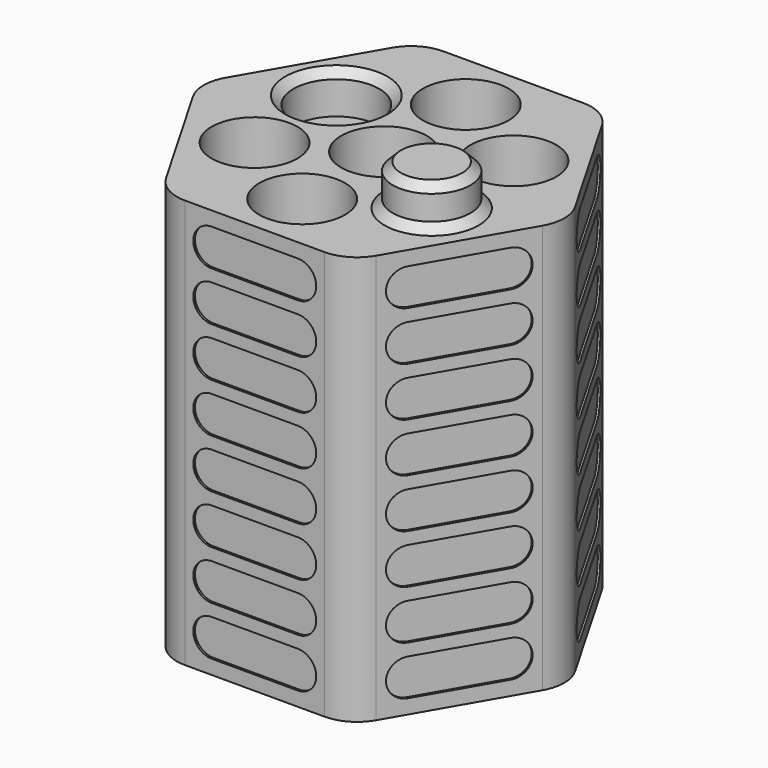
from build123d import *

# Parameters (mm, degrees)
F0_R      = 5.25
F0_R_2    = 4.75
F1_DEPTH  = 50
F2_DEPTH  = 5
F3_DEPTH  = 55
F4_DEPTH  = 45
F5_SIZE   = 1
F6_R      = 5
F8_DEPTH  = 0.25
F10_DEPTH = 0.25
F12_DEPTH = 0.25
F14_DEPTH = 0.25
F16_DEPTH = 0.25
F18_DEPTH = 0.25


with BuildPart() as f1:
    # F0 (on Top) → F1 (new body)
    with BuildSketch(Plane.XY):
        Polygon((11.4026678165, 19.75), (-11.4026678165, 19.75), (-22.805335633, 0), (-11.4026678165, -19.75), (11.4026678165, -19.75), (22.805335633, 0), align=None)
        with Locations((-10.8253175473, -6.25)):
            Circle(F0_R, mode=Mode.SUBTRACT)
        with Locations((0, -12.5)):
            Circle(F0_R, mode=Mode.SUBTRACT)
        with Locations((10.8253175473, -6.25)):
            Circle(F0_R_2, mode=Mode.SUBTRACT)
        with Locations((-10.8253175473, 6.25)):
            Circle(F0_R, mode=Mode.SUBTRACT)
        Circle(F0_R, mode=Mode.SUBTRACT)
        with Locations((10.8253175473, 6.25)):
            Circle(F0_R, mode=Mode.SUBTRACT)
        with Locations((0, 12.5)):
            Circle(F0_R, mode=Mode.SUBTRACT)
    extrude(amount=F1_DEPTH)

    # F0 (on Top) → F2 (join)
    with BuildSketch(Plane.XY):
        Circle(F0_R)
        with Locations((0, 12.5)):
            Circle(F0_R)
        with Locations((-10.8253175473, -6.25)):
            Circle(F0_R)
        with Locations((0, -12.5)):
            Circle(F0_R)
        with Locations((10.8253175473, 6.25)):
            Circle(F0_R)
    extrude(amount=F2_DEPTH)

    # F0 (on Top) → F3 (join)
    with BuildSketch(Plane.XY):
        with Locations((10.8253175473, -6.25)):
            Circle(F0_R_2)
    extrude(amount=F3_DEPTH)

    # F0 (on Top) → F4 (join)
    with BuildSketch(Plane.XY):
        with Locations((-10.8253175473, 6.25)):
            Circle(F0_R)
    extrude(amount=F4_DEPTH)

    # F5
    f5_edges = [f1.edges().sort_by_distance(p)[0] for p in [
        (6.075318, -6.25, 55),
        (-16.075318, 6.25, 50),
        (6.075318, -6.25, 50),
    ]]
    chamfer(f5_edges, length=F5_SIZE)

    # F6
    f6_edges = [f1.edges().sort_by_distance(p)[0] for p in [
        (22.805336, 0, 25),
        (11.402668, 19.75, 25),
        (-11.402668, 19.75, 25),
        (-22.805336, 0, 25),
        (-11.402668, -19.75, 25),
        (11.402668, -19.75, 25),
    ]]
    fillet(f6_edges, radius=F6_R)

    # F7 (on face) → F8 (cut)
    with BuildSketch(Plane.XZ.offset(19.75)):
        with BuildLine():
            Line((5.2659164705, 48.25), (-5.2659164705, 48.25))
            ThreePointArc((-5.2659164705, 48.25), (-7.5159164705, 46), (-5.2659164705, 43.75))
            Line((-5.2659164705, 43.75), (5.2659164705, 43.75))
            ThreePointArc((5.2659164705, 43.75), (7.5159164705, 46), (5.2659164705, 48.25))
        make_face()
        with BuildLine():
            Line((5.2659164705, 42.25), (-5.2659164705, 42.25))
            ThreePointArc((-5.2659164705, 42.25), (-7.5159164705, 40), (-5.2659164705, 37.75))
            Line((-5.2659164705, 37.75), (5.2659164705, 37.75))
            ThreePointArc((5.2659164705, 37.75), (7.5159164705, 40), (5.2659164705, 42.25))
        make_face()
        with BuildLine():
            Line((5.2659164705, 36.25), (-5.2659164705, 36.25))
            ThreePointArc((-5.2659164705, 36.25), (-7.5159164705, 34), (-5.2659164705, 31.75))
            Line((-5.2659164705, 31.75), (5.2659164705, 31.75))
            ThreePointArc((5.2659164705, 31.75), (7.5159164705, 34), (5.2659164705, 36.25))
        make_face()
        with BuildLine():
            Line((5.2659164705, 30.25), (-5.2659164705, 30.25))
            ThreePointArc((-5.2659164705, 30.25), (-7.5159164705, 28), (-5.2659164705, 25.75))
            Line((-5.2659164705, 25.75), (5.2659164705, 25.75))
            ThreePointArc((5.2659164705, 25.75), (7.5159164705, 28), (5.2659164705, 30.25))
        make_face()
        with BuildLine():
            Line((5.2659164705, 24.25), (-5.2659164705, 24.25))
            ThreePointArc((-5.2659164705, 24.25), (-7.5159164705, 22), (-5.2659164705, 19.75))
            Line((-5.2659164705, 19.75), (5.2659164705, 19.75))
            ThreePointArc((5.2659164705, 19.75), (7.5159164705, 22), (5.2659164705, 24.25))
        make_face()
        with BuildLine():
            Line((5.2659164705, 18.25), (-5.2659164705, 18.25))
            ThreePointArc((-5.2659164705, 18.25), (-7.5159164705, 16), (-5.2659164705, 13.75))
            Line((-5.2659164705, 13.75), (5.2659164705, 13.75))
            ThreePointArc((5.2659164705, 13.75), (7.5159164705, 16), (5.2659164705, 18.25))
        make_face()
        with BuildLine():
            Line((5.2659164705, 12.25), (-5.2659164705, 12.25))
            ThreePointArc((-5.2659164705, 12.25), (-7.5159164705, 10), (-5.2659164705, 7.75))
            Line((-5.2659164705, 7.75), (5.2659164705, 7.75))
            ThreePointArc((5.2659164705, 7.75), (7.5159164705, 10), (5.2659164705, 12.25))
        make_face()
        with BuildLine():
            Line((5.2659164705, 6.25), (-5.2659164705, 6.25))
            ThreePointArc((-5.2659164705, 6.25), (-7.5159164705, 4), (-5.2659164705, 1.75))
            Line((-5.2659164705, 1.75), (5.2659164705, 1.75))
            ThreePointArc((5.2659164705, 1.75), (7.5159164705, 4), (5.2659164705, 6.25))
        make_face()
    extrude(amount=-F8_DEPTH, mode=Mode.SUBTRACT)

    # F9 (on face) → F10 (cut)
    with BuildSketch(Plane(origin=(17.1040017247, -9.875, 0), x_dir=(0.5, 0.8660254038, 0), z_dir=(0.8660254038, -0.5, 0))):
        with BuildLine():
            Line((5.2659164705, 48.25), (-5.2659164705, 48.25))
            ThreePointArc((-5.2659164705, 48.25), (-7.5159164705, 46), (-5.2659164705, 43.75))
            Line((-5.2659164705, 43.75), (5.2659164705, 43.75))
            ThreePointArc((5.2659164705, 43.75), (7.5159164705, 46), (5.2659164705, 48.25))
        make_face()
        with BuildLine():
            Line((5.2659164705, 42.25), (-5.2659164705, 42.25))
            ThreePointArc((-5.2659164705, 42.25), (-7.5159164705, 40), (-5.2659164705, 37.75))
            Line((-5.2659164705, 37.75), (5.2659164705, 37.75))
            ThreePointArc((5.2659164705, 37.75), (7.5159164705, 40), (5.2659164705, 42.25))
        make_face()
        with BuildLine():
            Line((5.2659164705, 36.25), (-5.2659164705, 36.25))
            ThreePointArc((-5.2659164705, 36.25), (-7.5159164705, 34), (-5.2659164705, 31.75))
            Line((-5.2659164705, 31.75), (5.2659164705, 31.75))
            ThreePointArc((5.2659164705, 31.75), (7.5159164705, 34), (5.2659164705, 36.25))
        make_face()
        with BuildLine():
            Line((5.2659164705, 30.25), (-5.2659164705, 30.25))
            ThreePointArc((-5.2659164705, 30.25), (-7.5159164705, 28), (-5.2659164705, 25.75))
            Line((-5.2659164705, 25.75), (5.2659164705, 25.75))
            ThreePointArc((5.2659164705, 25.75), (7.5159164705, 28), (5.2659164705, 30.25))
        make_face()
        with BuildLine():
            Line((5.2659164705, 24.25), (-5.2659164705, 24.25))
            ThreePointArc((-5.2659164705, 24.25), (-7.5159164705, 22), (-5.2659164705, 19.75))
            Line((-5.2659164705, 19.75), (5.2659164705, 19.75))
            ThreePointArc((5.2659164705, 19.75), (7.5159164705, 22), (5.2659164705, 24.25))
        make_face()
        with BuildLine():
            Line((5.2659164705, 18.25), (-5.2659164705, 18.25))
            ThreePointArc((-5.2659164705, 18.25), (-7.5159164705, 16), (-5.2659164705, 13.75))
            Line((-5.2659164705, 13.75), (5.2659164705, 13.75))
            ThreePointArc((5.2659164705, 13.75), (7.5159164705, 16), (5.2659164705, 18.25))
        make_face()
        with BuildLine():
            Line((5.2659164705, 12.25), (-5.2659164705, 12.25))
            ThreePointArc((-5.2659164705, 12.25), (-7.5159164705, 10), (-5.2659164705, 7.75))
            Line((-5.2659164705, 7.75), (5.2659164705, 7.75))
            ThreePointArc((5.2659164705, 7.75), (7.5159164705, 10), (5.2659164705, 12.25))
        make_face()
        with BuildLine():
            Line((5.2659164705, 6.25), (-5.2659164705, 6.25))
            ThreePointArc((-5.2659164705, 6.25), (-7.5159164705, 4), (-5.2659164705, 1.75))
            Line((-5.2659164705, 1.75), (5.2659164705, 1.75))
            ThreePointArc((5.2659164705, 1.75), (7.5159164705, 4), (5.2659164705, 6.25))
        make_face()
    extrude(amount=-F10_DEPTH, mode=Mode.SUBTRACT)

    # F11 (on face) → F12 (cut)
    with BuildSketch(Plane(origin=(17.1040017247, 9.875, 0), x_dir=(-0.5, 0.8660254038, 0), z_dir=(0.8660254038, 0.5, 0))):
        with BuildLine():
            Line((5.2659164705, 48.25), (-5.2659164705, 48.25))
            ThreePointArc((-5.2659164705, 48.25), (-7.5159164705, 46), (-5.2659164705, 43.75))
            Line((-5.2659164705, 43.75), (5.2659164705, 43.75))
            ThreePointArc((5.2659164705, 43.75), (7.5159164705, 46), (5.2659164705, 48.25))
        make_face()
        with BuildLine():
            Line((5.2659164705, 42.25), (-5.2659164705, 42.25))
            ThreePointArc((-5.2659164705, 42.25), (-7.5159164705, 40), (-5.2659164705, 37.75))
            Line((-5.2659164705, 37.75), (5.2659164705, 37.75))
            ThreePointArc((5.2659164705, 37.75), (7.5159164705, 40), (5.2659164705, 42.25))
        make_face()
        with BuildLine():
            Line((5.2659164705, 36.25), (-5.2659164705, 36.25))
            ThreePointArc((-5.2659164705, 36.25), (-7.5159164705, 34), (-5.2659164705, 31.75))
            Line((-5.2659164705, 31.75), (5.2659164705, 31.75))
            ThreePointArc((5.2659164705, 31.75), (7.5159164705, 34), (5.2659164705, 36.25))
        make_face()
        with BuildLine():
            Line((5.2659164705, 30.25), (-5.2659164705, 30.25))
            ThreePointArc((-5.2659164705, 30.25), (-7.5159164705, 28), (-5.2659164705, 25.75))
            Line((-5.2659164705, 25.75), (5.2659164705, 25.75))
            ThreePointArc((5.2659164705, 25.75), (7.5159164705, 28), (5.2659164705, 30.25))
        make_face()
        with BuildLine():
            Line((5.2659164705, 24.25), (-5.2659164705, 24.25))
            ThreePointArc((-5.2659164705, 24.25), (-7.5159164705, 22), (-5.2659164705, 19.75))
            Line((-5.2659164705, 19.75), (5.2659164705, 19.75))
            ThreePointArc((5.2659164705, 19.75), (7.5159164705, 22), (5.2659164705, 24.25))
        make_face()
        with BuildLine():
            Line((5.2659164705, 18.25), (-5.2659164705, 18.25))
            ThreePointArc((-5.2659164705, 18.25), (-7.5159164705, 16), (-5.2659164705, 13.75))
            Line((-5.2659164705, 13.75), (5.2659164705, 13.75))
            ThreePointArc((5.2659164705, 13.75), (7.5159164705, 16), (5.2659164705, 18.25))
        make_face()
        with BuildLine():
            Line((5.2659164705, 12.25), (-5.2659164705, 12.25))
            ThreePointArc((-5.2659164705, 12.25), (-7.5159164705, 10), (-5.2659164705, 7.75))
            Line((-5.2659164705, 7.75), (5.2659164705, 7.75))
            ThreePointArc((5.2659164705, 7.75), (7.5159164705, 10), (5.2659164705, 12.25))
        make_face()
        with BuildLine():
            Line((5.2659164705, 6.25), (-5.2659164705, 6.25))
            ThreePointArc((-5.2659164705, 6.25), (-7.5159164705, 4), (-5.2659164705, 1.75))
            Line((-5.2659164705, 1.75), (5.2659164705, 1.75))
            ThreePointArc((5.2659164705, 1.75), (7.5159164705, 4), (5.2659164705, 6.25))
        make_face()
    extrude(amount=-F12_DEPTH, mode=Mode.SUBTRACT)

    # F13 (on face) → F14 (cut)
    with BuildSketch(Plane(origin=(0, 19.75, 0), x_dir=(-1, 0, 0), z_dir=(0, 1, 0))):
        with BuildLine():
            Line((5.2659164705, 48.25), (-5.2659164705, 48.25))
            ThreePointArc((-5.2659164705, 48.25), (-7.5159164705, 46), (-5.2659164705, 43.75))
            Line((-5.2659164705, 43.75), (5.2659164705, 43.75))
            ThreePointArc((5.2659164705, 43.75), (7.5159164705, 46), (5.2659164705, 48.25))
        make_face()
        with BuildLine():
            Line((5.2659164705, 42.25), (-5.2659164705, 42.25))
            ThreePointArc((-5.2659164705, 42.25), (-7.5159164705, 40), (-5.2659164705, 37.75))
            Line((-5.2659164705, 37.75), (5.2659164705, 37.75))
            ThreePointArc((5.2659164705, 37.75), (7.5159164705, 40), (5.2659164705, 42.25))
        make_face()
        with BuildLine():
            Line((5.2659164705, 36.25), (-5.2659164705, 36.25))
            ThreePointArc((-5.2659164705, 36.25), (-7.5159164705, 34), (-5.2659164705, 31.75))
            Line((-5.2659164705, 31.75), (5.2659164705, 31.75))
            ThreePointArc((5.2659164705, 31.75), (7.5159164705, 34), (5.2659164705, 36.25))
        make_face()
        with BuildLine():
            Line((5.2659164705, 30.25), (-5.2659164705, 30.25))
            ThreePointArc((-5.2659164705, 30.25), (-7.5159164705, 28), (-5.2659164705, 25.75))
            Line((-5.2659164705, 25.75), (5.2659164705, 25.75))
            ThreePointArc((5.2659164705, 25.75), (7.5159164705, 28), (5.2659164705, 30.25))
        make_face()
        with BuildLine():
            Line((5.2659164705, 24.25), (-5.2659164705, 24.25))
            ThreePointArc((-5.2659164705, 24.25), (-7.5159164705, 22), (-5.2659164705, 19.75))
            Line((-5.2659164705, 19.75), (5.2659164705, 19.75))
            ThreePointArc((5.2659164705, 19.75), (7.5159164705, 22), (5.2659164705, 24.25))
        make_face()
        with BuildLine():
            Line((5.2659164705, 18.25), (-5.2659164705, 18.25))
            ThreePointArc((-5.2659164705, 18.25), (-7.5159164705, 16), (-5.2659164705, 13.75))
            Line((-5.2659164705, 13.75), (5.2659164705, 13.75))
            ThreePointArc((5.2659164705, 13.75), (7.5159164705, 16), (5.2659164705, 18.25))
        make_face()
        with BuildLine():
            Line((5.2659164705, 12.25), (-5.2659164705, 12.25))
            ThreePointArc((-5.2659164705, 12.25), (-7.5159164705, 10), (-5.2659164705, 7.75))
            Line((-5.2659164705, 7.75), (5.2659164705, 7.75))
            ThreePointArc((5.2659164705, 7.75), (7.5159164705, 10), (5.2659164705, 12.25))
        make_face()
        with BuildLine():
            Line((5.2659164705, 6.25), (-5.2659164705, 6.25))
            ThreePointArc((-5.2659164705, 6.25), (-7.5159164705, 4), (-5.2659164705, 1.75))
            Line((-5.2659164705, 1.75), (5.2659164705, 1.75))
            ThreePointArc((5.2659164705, 1.75), (7.5159164705, 4), (5.2659164705, 6.25))
        make_face()
    extrude(amount=-F14_DEPTH, mode=Mode.SUBTRACT)

    # F15 (on face) → F16 (cut)
    with BuildSketch(Plane(origin=(-17.1040017247, 9.875, 0), x_dir=(-0.5, -0.8660254038, 0), z_dir=(-0.8660254038, 0.5, 0))):
        with BuildLine():
            Line((5.2659164705, 48.25), (-5.2659164705, 48.25))
            ThreePointArc((-5.2659164705, 48.25), (-7.5159164705, 46), (-5.2659164705, 43.75))
            Line((-5.2659164705, 43.75), (5.2659164705, 43.75))
            ThreePointArc((5.2659164705, 43.75), (7.5159164705, 46), (5.2659164705, 48.25))
        make_face()
        with BuildLine():
            Line((5.2659164705, 42.25), (-5.2659164705, 42.25))
            ThreePointArc((-5.2659164705, 42.25), (-7.5159164705, 40), (-5.2659164705, 37.75))
            Line((-5.2659164705, 37.75), (5.2659164705, 37.75))
            ThreePointArc((5.2659164705, 37.75), (7.5159164705, 40), (5.2659164705, 42.25))
        make_face()
        with BuildLine():
            Line((5.2659164705, 36.25), (-5.2659164705, 36.25))
            ThreePointArc((-5.2659164705, 36.25), (-7.5159164705, 34), (-5.2659164705, 31.75))
            Line((-5.2659164705, 31.75), (5.2659164705, 31.75))
            ThreePointArc((5.2659164705, 31.75), (7.5159164705, 34), (5.2659164705, 36.25))
        make_face()
        with BuildLine():
            Line((5.2659164705, 30.25), (-5.2659164705, 30.25))
            ThreePointArc((-5.2659164705, 30.25), (-7.5159164705, 28), (-5.2659164705, 25.75))
            Line((-5.2659164705, 25.75), (5.2659164705, 25.75))
            ThreePointArc((5.2659164705, 25.75), (7.5159164705, 28), (5.2659164705, 30.25))
        make_face()
        with BuildLine():
            Line((5.2659164705, 24.25), (-5.2659164705, 24.25))
            ThreePointArc((-5.2659164705, 24.25), (-7.5159164705, 22), (-5.2659164705, 19.75))
            Line((-5.2659164705, 19.75), (5.2659164705, 19.75))
            ThreePointArc((5.2659164705, 19.75), (7.5159164705, 22), (5.2659164705, 24.25))
        make_face()
        with BuildLine():
            Line((5.2659164705, 18.25), (-5.2659164705, 18.25))
            ThreePointArc((-5.2659164705, 18.25), (-7.5159164705, 16), (-5.2659164705, 13.75))
            Line((-5.2659164705, 13.75), (5.2659164705, 13.75))
            ThreePointArc((5.2659164705, 13.75), (7.5159164705, 16), (5.2659164705, 18.25))
        make_face()
        with BuildLine():
            Line((5.2659164705, 12.25), (-5.2659164705, 12.25))
            ThreePointArc((-5.2659164705, 12.25), (-7.5159164705, 10), (-5.2659164705, 7.75))
            Line((-5.2659164705, 7.75), (5.2659164705, 7.75))
            ThreePointArc((5.2659164705, 7.75), (7.5159164705, 10), (5.2659164705, 12.25))
        make_face()
        with BuildLine():
            Line((5.2659164705, 6.25), (-5.2659164705, 6.25))
            ThreePointArc((-5.2659164705, 6.25), (-7.5159164705, 4), (-5.2659164705, 1.75))
            Line((-5.2659164705, 1.75), (5.2659164705, 1.75))
            ThreePointArc((5.2659164705, 1.75), (7.5159164705, 4), (5.2659164705, 6.25))
        make_face()
    extrude(amount=-F16_DEPTH, mode=Mode.SUBTRACT)

    # F17 (on face) → F18 (cut)
    with BuildSketch(Plane(origin=(-17.1040017247, -9.875, 0), x_dir=(0.5, -0.8660254038, 0), z_dir=(-0.8660254038, -0.5, 0))):
        with BuildLine():
            Line((5.2659164705, 48.25), (-5.2659164705, 48.25))
            ThreePointArc((-5.2659164705, 48.25), (-7.5159164705, 46), (-5.2659164705, 43.75))
            Line((-5.2659164705, 43.75), (5.2659164705, 43.75))
            ThreePointArc((5.2659164705, 43.75), (7.5159164705, 46), (5.2659164705, 48.25))
        make_face()
        with BuildLine():
            Line((5.2659164705, 42.25), (-5.2659164705, 42.25))
            ThreePointArc((-5.2659164705, 42.25), (-7.5159164705, 40), (-5.2659164705, 37.75))
            Line((-5.2659164705, 37.75), (5.2659164705, 37.75))
            ThreePointArc((5.2659164705, 37.75), (7.5159164705, 40), (5.2659164705, 42.25))
        make_face()
        with BuildLine():
            Line((5.2659164705, 36.25), (-5.2659164705, 36.25))
            ThreePointArc((-5.2659164705, 36.25), (-7.5159164705, 34), (-5.2659164705, 31.75))
            Line((-5.2659164705, 31.75), (5.2659164705, 31.75))
            ThreePointArc((5.2659164705, 31.75), (7.5159164705, 34), (5.2659164705, 36.25))
        make_face()
        with BuildLine():
            Line((5.2659164705, 30.25), (-5.2659164705, 30.25))
            ThreePointArc((-5.2659164705, 30.25), (-7.5159164705, 28), (-5.2659164705, 25.75))
            Line((-5.2659164705, 25.75), (5.2659164705, 25.75))
            ThreePointArc((5.2659164705, 25.75), (7.5159164705, 28), (5.2659164705, 30.25))
        make_face()
        with BuildLine():
            Line((5.2659164705, 24.25), (-5.2659164705, 24.25))
            ThreePointArc((-5.2659164705, 24.25), (-7.5159164705, 22), (-5.2659164705, 19.75))
            Line((-5.2659164705, 19.75), (5.2659164705, 19.75))
            ThreePointArc((5.2659164705, 19.75), (7.5159164705, 22), (5.2659164705, 24.25))
        make_face()
        with BuildLine():
            Line((5.2659164705, 18.25), (-5.2659164705, 18.25))
            ThreePointArc((-5.2659164705, 18.25), (-7.5159164705, 16), (-5.2659164705, 13.75))
            Line((-5.2659164705, 13.75), (5.2659164705, 13.75))
            ThreePointArc((5.2659164705, 13.75), (7.5159164705, 16), (5.2659164705, 18.25))
        make_face()
        with BuildLine():
            Line((5.2659164705, 12.25), (-5.2659164705, 12.25))
            ThreePointArc((-5.2659164705, 12.25), (-7.5159164705, 10), (-5.2659164705, 7.75))
            Line((-5.2659164705, 7.75), (5.2659164705, 7.75))
            ThreePointArc((5.2659164705, 7.75), (7.5159164705, 10), (5.2659164705, 12.25))
        make_face()
        with BuildLine():
            Line((5.2659164705, 6.25), (-5.2659164705, 6.25))
            ThreePointArc((-5.2659164705, 6.25), (-7.5159164705, 4), (-5.2659164705, 1.75))
            Line((-5.2659164705, 1.75), (5.2659164705, 1.75))
            ThreePointArc((5.2659164705, 1.75), (7.5159164705, 4), (5.2659164705, 6.25))
        make_face()
    extrude(amount=-F18_DEPTH, mode=Mode.SUBTRACT)


solid = f1.part
